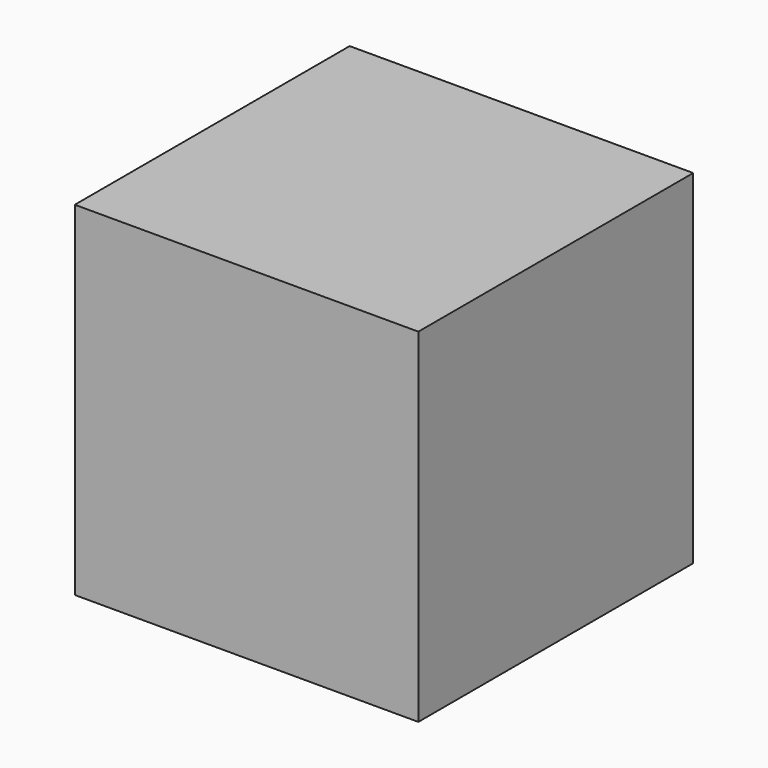
from build123d import *

# Parameters (mm, degrees)
F0_W     = 30
F0_H     = 30
F1_DEPTH = 30


# Not quite as in the source:
# - a feature names something its author has since deleted; it is built from what else it names


with BuildPart() as f1:
    # F0 (on Top) → F1 (new body)
    with BuildSketch(Plane.XY):
        Rectangle(F0_W, F0_H)
    extrude(amount=F1_DEPTH)


solid = f1.part
